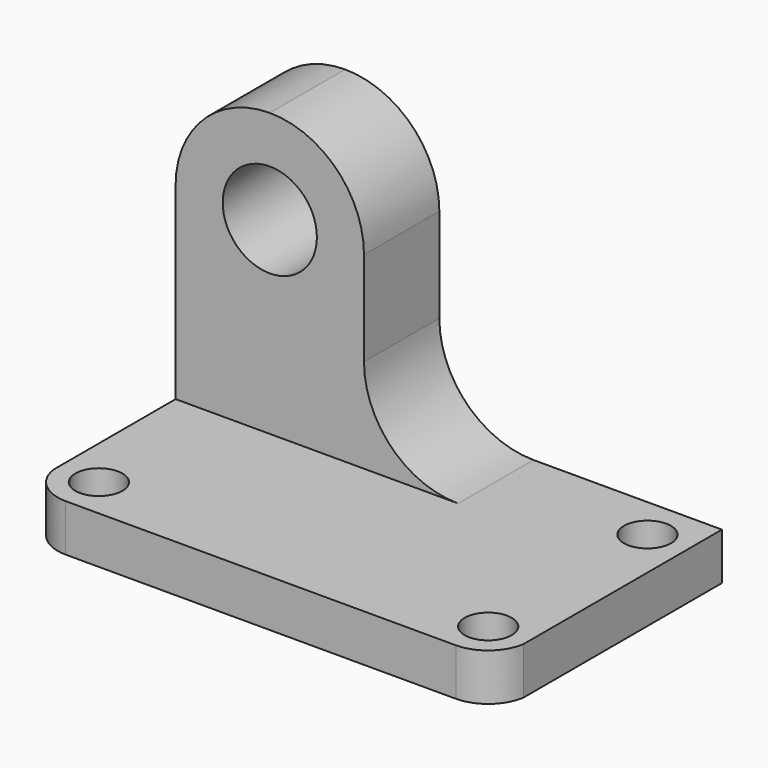
from build123d import *

# Parameters (mm, degrees)
F0_W      = 63.5
F0_H      = 44.45
F1_DEPTH  = 38.1
F2_W      = 25.4
F2_H      = 38.1
F3_DEPTH  = 63.5
F4_W      = 25.4
F4_H      = 38.1
F5_DEPTH  = 12.7
F7_DEPTH  = 12.7
F9_DEPTH  = 12.7
F10_R     = 6.35
F11_DEPTH = 12.7
F13_DEPTH = 6.35
F14_R     = 3.175
F15_DEPTH = 6.35


with BuildPart() as f1:
    # F0 (on Front) → F1 (new body)
    with BuildSketch(Plane.XZ):
        with Locations((-34.4360737465, 22.225)):
            Rectangle(F0_W, F0_H)
    extrude(amount=F1_DEPTH)

    # F2 (on face) → F3 (cut)
    with BuildSketch(Plane(origin=(-66.1860737465, 0, 0), x_dir=(0, -1, 0), z_dir=(-1, 0, 0))):
        with Locations((25.4, 25.4)):
            Rectangle(F2_W, F2_H)
    extrude(amount=-F3_DEPTH, mode=Mode.SUBTRACT)

    # F4 (on face) → F5 (cut)
    with BuildSketch(Plane.XZ.offset(12.7)):
        with Locations((-15.3860737465, 25.4)):
            Rectangle(F4_W, F4_H)
    extrude(amount=-F5_DEPTH, mode=Mode.SUBTRACT)

    # F6 (on face) → F7 (cut)
    with BuildSketch(Plane.XZ.offset(12.7)):
        with BuildLine():
            Line((-40.7860737465, 44.45), (-40.7860737465, 19.05))
            ThreePointArc((-40.7860737465, 19.05), (-37.0663298676, 10.0697438789), (-28.0860737465, 6.35))
            Line((-28.0860737465, 6.35), (-28.0860737465, 44.45))
            Line((-28.0860737465, 44.45), (-40.7860737465, 44.45))
        make_face()
    extrude(amount=-F7_DEPTH, mode=Mode.SUBTRACT)

    # F8 (on face) → F9 (cut)
    with BuildSketch(Plane.XZ.offset(12.7)):
        with BuildLine():
            ThreePointArc((-53.4860737465, 44.45), (-44.5058176254, 40.7302561211), (-40.7860737465, 31.75))
            Line((-40.7860737465, 31.75), (-40.7860737465, 44.45))
            Line((-40.7860737465, 44.45), (-53.4860737465, 44.45))
        make_face()
        with BuildLine():
            ThreePointArc((-66.1860737465, 31.75), (-62.4663298676, 40.7302561211), (-53.4860737465, 44.45))
            Line((-53.4860737465, 44.45), (-66.1860737465, 44.45))
            Line((-66.1860737465, 44.45), (-66.1860737465, 31.75))
        make_face()
    extrude(amount=-F9_DEPTH, mode=Mode.SUBTRACT)

    # F10 (on face) → F11 (cut)
    with BuildSketch(Plane.XZ.offset(12.7)):
        with Locations((-53.4860737465, 31.75)):
            Circle(F10_R)
    extrude(amount=-F11_DEPTH, mode=Mode.SUBTRACT)

    # F12 (on face) → F13 (cut)
    with BuildSketch(Plane.XY.offset(6.35)):
        with BuildLine():
            ThreePointArc((-60.6986656785, -38.1), (-64.3552084633, -36.6998783466), (-66.1860737465, -33.238870098))
            Line((-66.1860737465, -33.238870098), (-66.1860737465, -38.1))
            Line((-66.1860737465, -38.1), (-60.6986656785, -38.1))
        make_face()
        with BuildLine():
            ThreePointArc((-2.6860737465, -33.4266640174), (-4.5022022533, -36.7506081509), (-8.0414209515, -38.1))
            Line((-8.0414209515, -38.1), (-2.6860737465, -38.1))
            Line((-2.6860737465, -38.1), (-2.6860737465, -33.4266640174))
        make_face()
    extrude(amount=-F13_DEPTH, mode=Mode.SUBTRACT)

    # F14 (on face) → F15 (cut)
    with BuildSketch(Plane.XY.offset(6.35)):
        with Locations((-60.6629240595, -32.5319026628)):
            Circle(F14_R)
        with Locations((-8.1017104419, -32.6257996225)):
            Circle(F14_R)
        with Locations((-8.1017104419, -5.7779387571)):
            Circle(F14_R)
    extrude(amount=-F15_DEPTH, mode=Mode.SUBTRACT)


solid = f1.part
